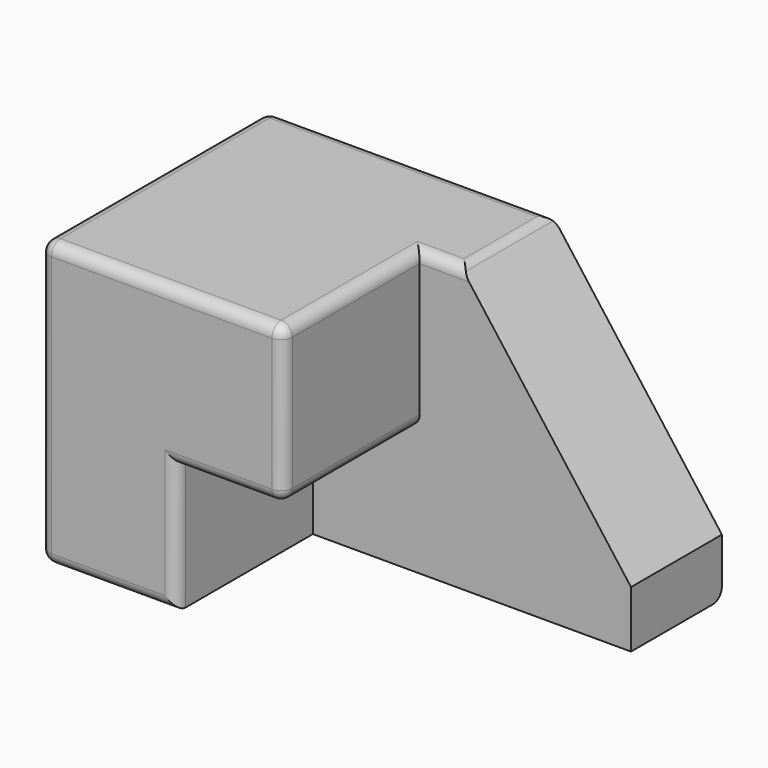
from build123d import *

# Parameters (mm, degrees)
F0_W     = 203.2
F0_H     = 127
F1_DEPTH = 127
F3_DEPTH = 76.2
F4_SIZE2 = 101.6
F4_SIZE  = 76.2
F5_R     = 5.08


# Not quite as in the source:
# - the program builds the solid bodies; features that only make, move or delete a surface that nothing else refers to are left out


with BuildPart() as f1:
    # F0 (on Front) → F1 (new body)
    with BuildSketch(Plane.XZ):
        Rectangle(F0_W, F0_H)
    extrude(amount=F1_DEPTH)

    # F2 (on face) → F3 (cut)
    with BuildSketch(Plane.XZ.offset(127)):
        Polygon((-40.63635692, -6.0839741491), (-40.63635692, -63.5), (101.6, -63.5), (101.6, 63.5), (7.1171009913, 63.5), (7.1171009913, -6.0839741491), align=None)
    extrude(amount=-F3_DEPTH, mode=Mode.SUBTRACT)

    # F4
    f4_edges = [f1.edges().sort_by_distance(p)[0] for p in [
        (101.6, -25.4, 63.5),
    ]]
    f4_side = f1.faces().sort_by_distance((-21.033148, -53.671887, 63.5))[0]
    chamfer(f4_edges, length=F4_SIZE, length2=F4_SIZE2, reference=f4_side)

    # F5
    f5_edges = [f1.edges().sort_by_distance(p)[0] for p in [
        (-47.24145, -127, 63.5),
        (7.117101, -127, 28.708013),
        (7.117101, -88.9, -6.083974),
        (7.117101, -88.9, 63.5),
        (16.25855, -50.8, 63.5),
        (25.4, -25.4, 63.5),
        (-16.759628, -127, -6.083974),
        (-40.636357, -127, -34.791987),
        (-71.118178, -127, -63.5),
        (-101.6, -127, 0),
        (-101.6, -63.5, 63.5),
        (-101.6, -63.5, -63.5),
        (-101.6, 0, 0),
        (-38.1, 0, 63.5),
        (0, 0, -63.5),
    ]]
    fillet(f5_edges, radius=F5_R)


solid = f1.part
